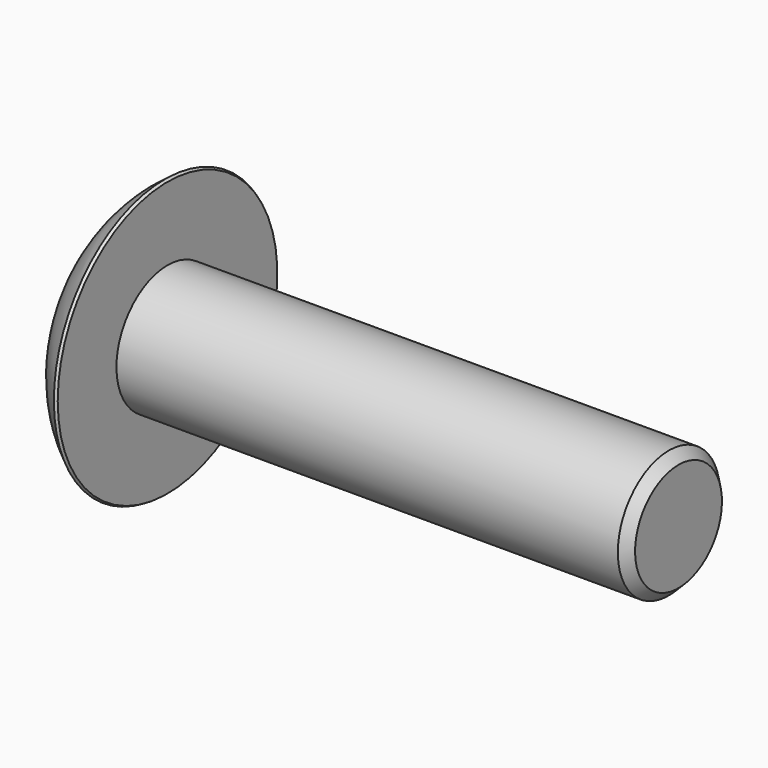
from build123d import *

# Parameters (mm, degrees)
F0_W     = 40
F0_H     = 5
F2_SIZE  = 0.75
F3_R     = 11
F3_R_2   = 5
F4_DEPTH = 5
F7_W     = 5
F7_H     = 4
F8_DEPTH = 12.5


# Not quite as in the source:
# - a fillet or chamfer that OpenCascade refuses, or shapes differently, is made with other operations: its cross-section is extruded or revolved along the edge and cut away or added


with BuildPart() as f1:
    # F0 (on Front) → F1 (revolve)
    with BuildSketch(Plane.XZ):
        with Locations((0, 2.5)):
            Rectangle(F0_W, F0_H)
    revolve(axis=Axis((0, 0, 0), (1, 0, 0)))

    # F2
    f2_edges = [f1.edges().sort_by_distance(p)[0] for p in [
        (20, 0, -5),
    ]]
    chamfer(f2_edges, length=F2_SIZE)

    # F3 (on face) → F4 (join)
    with BuildSketch(Plane(origin=(-20, 0, 0), x_dir=(0, -1, 0), z_dir=(-1, 0, 0))):
        Circle(F3_R)
        Circle(F3_R_2, mode=Mode.SUBTRACT)
        Circle(F3_R_2)
    extrude(amount=F4_DEPTH)

    # F5: fillet of radius 11 on 1 edges, made by hand

    # F5_s1 → F5_t2 (revolve, cut)
    with BuildSketch(Plane.XY):
        with BuildLine():
            ThreePointArc((-20, -11), (-23.6695398029, -7.0244997836), (-25, -1.7804555427))
            Line((-25, -1.7804555427), (-25, -11))
            Line((-25, -11), (-20, -11))
        make_face()
    revolve(axis=Axis((-25, 0, 0), (-1, 0, 0)), mode=Mode.SUBTRACT)

    # F6: chamfer of 0.25 on 1 edges, made by hand

    # F6_s1 → F6_t2 (revolve, cut)
    with BuildSketch(Plane.XY):
        with BuildLine():
            Line((-19.9911548293, -10.7418502329), (-20.2209951465, -10.8630715284))
            Line((-20.2209951465, -10.8630715284), (-20.2238188511, -10.8671978697))
            ThreePointArc((-20.2238188511, -10.8671978697), (-20.1112438047, -10.9326533203), (-20.0027272727, -11.004190702))
            Line((-20.0027272727, -11.004190702), (-19.995, -11))
            ThreePointArc((-19.995, -11), (-19.995, -10.8709251165), (-19.9861548293, -10.7418502329))
            Line((-19.9861548293, -10.7418502329), (-19.9911548293, -10.7418502329))
        make_face()
    revolve(axis=Axis((-20, 0, 0), (-1, 0, 0)), mode=Mode.SUBTRACT)

    # F7 (on Top) → F8 (cut, symmetric)
    with BuildSketch(Plane.XY):
        with Locations((-25.2117160708, 0)):
            Rectangle(F7_W, F7_H)
    extrude(amount=F8_DEPTH, both=True, mode=Mode.SUBTRACT)


solid = f1.part
